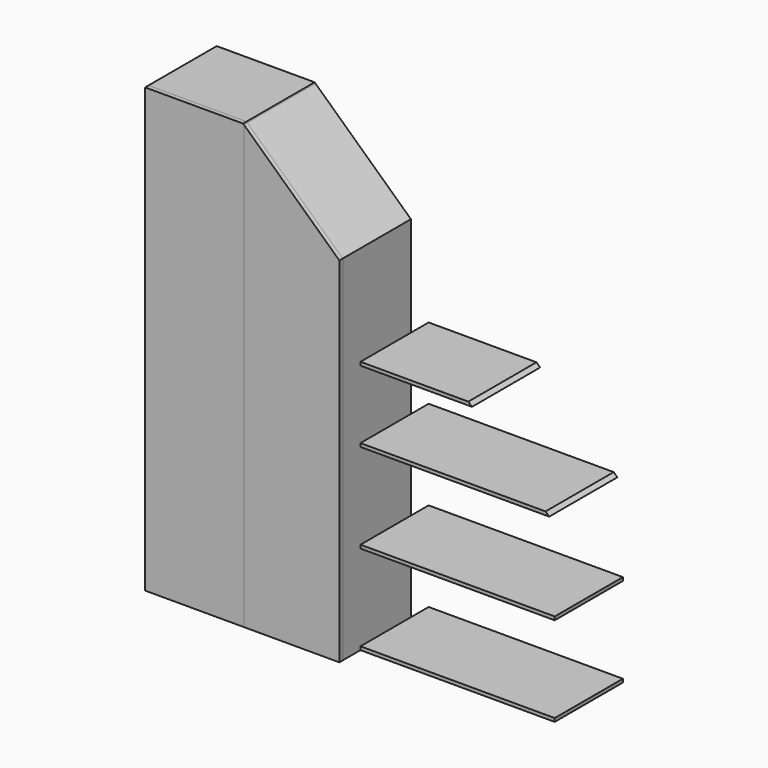
from build123d import *

# Parameters (mm, degrees)
F0_W     = 540
F0_H     = 310
F0_H_2   = 280
F0_H_3   = 260
F0_H_4   = 20
F1_DEPTH = 500
F0_H_5   = 920
F0_H_6   = 275
F0_H_7   = 35
F0_H_8   = 30
F2_DEPTH = 25
F0_H_9   = 250
F0_H_10  = 230
F3_DEPTH = 25
F4_START = -130
F4_DEPTH = 500
F0_W_2   = 1140
F0_H_11  = 20.0000000002


# Not quite as in the source:
# - a feature names something its author has since deleted; it is built from what else it names


with BuildPart() as f1:
    # F0 (on Front) → F1 (new body)
    with BuildSketch(Plane.XZ):
        Polygon((-1140, -1300), (-560, -1300), (-560, -1280), (-560, -1050), (-560, -800), (-560, -550), (-560, -530), (-560, -220), (-560, -200), (-560, 110), (-560, 130), (-560, 440), (-560, 460), (-560, 770), (-560, 790), (-560, 1268.0993919815), (-560, 1295.366568915), (-565, 1300), (-1140, 1300), align=None)
        with Locations((-850, -1125)):
            Rectangle(F0_W, F0_H, mode=Mode.SUBTRACT)
        with Locations((-850, -795)):
            Rectangle(F0_W, F0_H, mode=Mode.SUBTRACT)
        Polygon((-580, -290), (-580, -325), (-580, -345), (-580, -620), (-1120, -620), (-1120, -345), (-1120, -325), (-1120, -290), align=None, mode=Mode.SUBTRACT)
        Polygon((-1120, 700), (-580, 700), (-580, 670), (-580, 650), (-580, -270), (-1120, -270), (-1120, 650), (-1120, 670), align=None, mode=Mode.SUBTRACT)
        with Locations((-850, 860)):
            Rectangle(F0_W, F0_H_2, mode=Mode.SUBTRACT)
        with Locations((-850, 1150)):
            Rectangle(F0_W, F0_H_3, mode=Mode.SUBTRACT)
        Polygon((-20.0000000001, -250), (0, -250), (0, -230), (0, 170), (0, 190), (0, 776.4222873899), (-560, 1295.366568915), (-560, 1268.0993919815), (-44.0762890327, 790), (-560, 790), (-560, 770), (-22.4940105517, 770), (-20, 767.6888347967), (-20, 720), (-20, 700), (-20, 460), (-560, 460), (-560, 440), (-20, 440), (-20, 374.9999928474), (-20, 354.9999928474), (-20, 130), (-20, 110), (-20, -200), (-560, -200), (-560, -220), (-20, -220), align=None)
        with Locations((-290, 120)):
            Rectangle(F0_W, F0_H_4)
        Polygon((-560, -1300), (0, -1300), (0, -1280), (0, -775), (0, -755), (0, -250), (-20.0000000001, -250), (-20, -285.0000071528), (-20, -305.0000071528), (-20, -530), (-560, -530), (-560, -550), (-20, -550), (-20, -800), (-20, -1050), (-20, -1280), (-560, -1280), align=None)
    extrude(amount=-F1_DEPTH)


with BuildPart() as f2:
    # F0 (on Front) → F2 (new body)
    with BuildSketch(Plane.XZ):
        Polygon((-1140, -1300), (-560, -1300), (-560, -1280), (-560, -1050), (-560, -800), (-560, -550), (-560, -530), (-560, -220), (-560, -200), (-560, 110), (-560, 130), (-560, 440), (-560, 460), (-560, 770), (-560, 790), (-560, 1268.0993919815), (-560, 1295.366568915), (-565, 1300), (-1140, 1300), align=None)
        with Locations((-850, -1125)):
            Rectangle(F0_W, F0_H, mode=Mode.SUBTRACT)
        with Locations((-850, -795)):
            Rectangle(F0_W, F0_H, mode=Mode.SUBTRACT)
        Polygon((-580, -290), (-580, -325), (-580, -345), (-580, -620), (-1120, -620), (-1120, -345), (-1120, -325), (-1120, -290), align=None, mode=Mode.SUBTRACT)
        Polygon((-1120, 700), (-580, 700), (-580, 670), (-580, 650), (-580, -270), (-1120, -270), (-1120, 650), (-1120, 670), align=None, mode=Mode.SUBTRACT)
        with Locations((-850, 860)):
            Rectangle(F0_W, F0_H_2, mode=Mode.SUBTRACT)
        with Locations((-850, 1150)):
            Rectangle(F0_W, F0_H_3, mode=Mode.SUBTRACT)
        with Locations((-850, 190)):
            Rectangle(F0_W, F0_H_5)
        with Locations((-850, -795)):
            Rectangle(F0_W, F0_H)
        with Locations((-850, -1125)):
            Rectangle(F0_W, F0_H)
        with Locations((-850, 860)):
            Rectangle(F0_W, F0_H_2)
        with Locations((-850, -482.5)):
            Rectangle(F0_W, F0_H_6)
        with Locations((-850, 1150)):
            Rectangle(F0_W, F0_H_3)
        with Locations((-850, -307.5)):
            Rectangle(F0_W, F0_H_7)
        with Locations((-850, 685)):
            Rectangle(F0_W, F0_H_8)
        with Locations((-850, 660)):
            Rectangle(F0_W, F0_H_4)
        with Locations((-850, -335)):
            Rectangle(F0_W, F0_H_4)
    extrude(amount=F2_DEPTH)


with BuildPart() as f3:
    # F0 (on Front) → F3 (new body)
    with BuildSketch(Plane.XZ):
        Polygon((-44.0762890327, 790), (-560, 1268.0993919815), (-560, 790), align=None)
        Polygon((-560, -1300), (0, -1300), (0, -1280), (0, -775), (0, -755), (0, -250), (-20.0000000001, -250), (-20, -285.0000071528), (-20, -305.0000071528), (-20, -530), (-560, -530), (-560, -550), (-20, -550), (-20, -800), (-20, -1050), (-20, -1280), (-560, -1280), align=None)
        with Locations((-290, -675)):
            Rectangle(F0_W, F0_H_9)
        with Locations((-290, -925)):
            Rectangle(F0_W, F0_H_9)
        with Locations((-290, -1165)):
            Rectangle(F0_W, F0_H_10)
        Polygon((-20, -285.0000071528), (-20, -250), (-20, -220), (-560, -220), (-560, -530), (-20, -530), (-20, -305.0000071528), align=None)
        Polygon((-20.0000000001, -250), (0, -250), (0, -230), (0, 170), (0, 190), (0, 776.4222873899), (-560, 1295.366568915), (-560, 1268.0993919815), (-44.0762890327, 790), (-560, 790), (-560, 770), (-22.4940105517, 770), (-20, 767.6888347967), (-20, 720), (-20, 700), (-20, 460), (-560, 460), (-560, 440), (-20, 440), (-20, 374.9999928474), (-20, 354.9999928474), (-20, 130), (-20, 110), (-20, -200), (-560, -200), (-560, -220), (-20, -220), align=None)
        with Locations((-290, -45)):
            Rectangle(F0_W, F0_H)
        with Locations((-290, 120)):
            Rectangle(F0_W, F0_H_4)
        Polygon((-20, 440), (-560, 440), (-560, 130), (-20, 130), (-20, 354.9999928474), (-20, 374.9999928474), align=None)
        Polygon((-22.4940105517, 770), (-560, 770), (-560, 460), (-20, 460), (-20, 700), (-20, 720), (-20, 767.6888347967), align=None)
    extrude(amount=F3_DEPTH)


with BuildPart() as f4:
    # F0 (on Front) → F4 (new body)
    with BuildSketch(Plane.XZ.offset(F4_START)):
        Polygon((0, 190), (0, 170), (654.3987341771, 169.9999999999), (632.8164556961, 189.9999999999), align=None)
    extrude(amount=-F4_DEPTH)


with BuildPart() as f4b:
    # F0 (on Front) → F4, piece 2 (new body)
    with BuildSketch(Plane.XZ.offset(F4_START)):
        Polygon((0, -230), (0, -250), (1107.6265822783, -250.0000000001), (1086.0443037973, -230.0000000001), align=None)
    extrude(amount=-F4_DEPTH)


with BuildPart() as f4c:
    # F0 (on Front) → F4, piece 3 (new body)
    with BuildSketch(Plane.XZ.offset(F4_START)):
        with Locations((570, -765.0000000001)):
            Rectangle(F0_W_2, F0_H_11)
    extrude(amount=-F4_DEPTH)


with BuildPart() as f4d:
    # F0 (on Front) → F4, piece 4 (new body)
    with BuildSketch(Plane.XZ.offset(F4_START)):
        with Locations((570, -1290)):
            Rectangle(F0_W_2, F0_H_4)
    extrude(amount=-F4_DEPTH)


solid = Compound([f1.part, f2.part, f3.part, f4.part, f4b.part, f4c.part, f4d.part])
